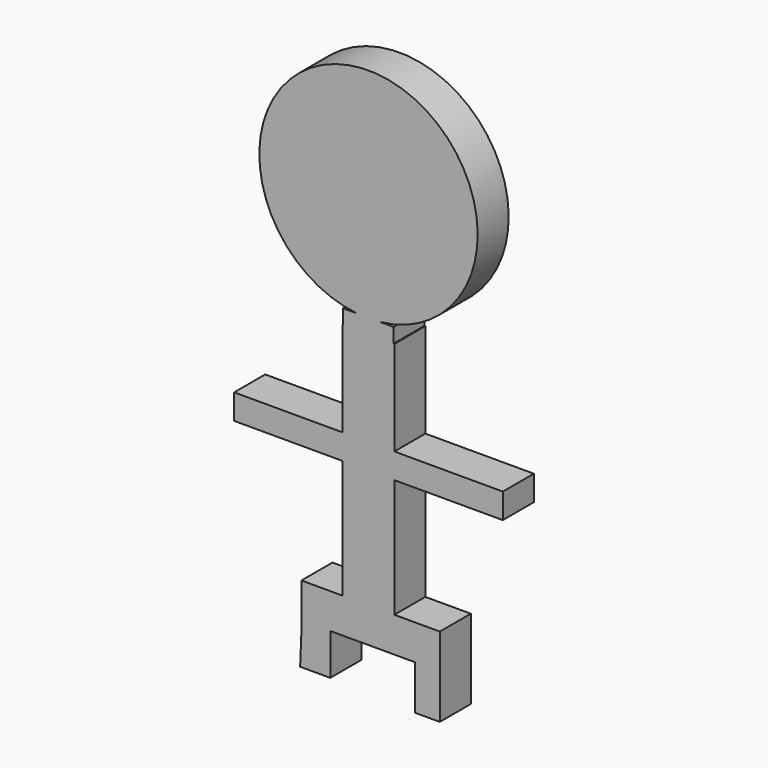
from build123d import *

# Parameters (mm, degrees)
F0_R      = 71.5350962672
F1_DEPTH  = 25.4
F4_W      = 16.7800951749
F4_H      = 74.4879245758
F4_W_2    = 16.4273940027
F5_DEPTH  = 25.4
F6_W      = 176.0196238756
F6_H      = 16.4934694767
F7_DEPTH  = 25.4
F8_W      = 33.9048393071
F8_H      = 156.475931406
F9_DEPTH  = 25.4
F11_DEPTH = 25.4


# Not quite as in the source:
# - the program builds the solid bodies; features that only make, move or delete a surface that nothing else refers to are left out


with BuildPart() as f1:
    # F0 (on Front) → F1 (new body)
    with BuildSketch(Plane.XZ):
        Circle(F0_R)
    extrude(amount=F1_DEPTH)

    # F4 (on Front) → F5 (join)
    with BuildSketch(Plane.XZ):
        with Locations((-8.3900475875, -108.3736568689)):
            Rectangle(F4_W, F4_H)
        with Locations((8.2136970013, -108.3736568689)):
            Rectangle(F4_W_2, F4_H)
    extrude(amount=F5_DEPTH)

    # F6 (on Front) → F7 (join)
    with BuildSketch(Plane.XZ):
        with Locations((0, -151.0558873415)):
            Rectangle(F6_W, F6_H)
    extrude(amount=F7_DEPTH)

    # F8 (on Front) → F9 (join)
    with BuildSketch(Plane.XZ):
        with Locations((0, -158.9946001768)):
            Rectangle(F8_W, F8_H)
    extrude(amount=F9_DEPTH)

    # F10 (on Front) → F11 (join)
    with BuildSketch(Plane.XZ):
        Polygon((46.7250607908, -236.9969040155), (0, -236.9969040155), (-43.9401827753, -236.9969040155), (-43.9401827753, -266.2233710289), (-44.8115989566, -287.0510220528), (-25.0311624259, -287.0510220528), (-25.0311624259, -259.9867582321), (30.4474048316, -259.9867582321), (30.4474048316, -289.1219854355), (46.7250607908, -289.1219854355), align=None)
    extrude(amount=F11_DEPTH)


solid = f1.part
